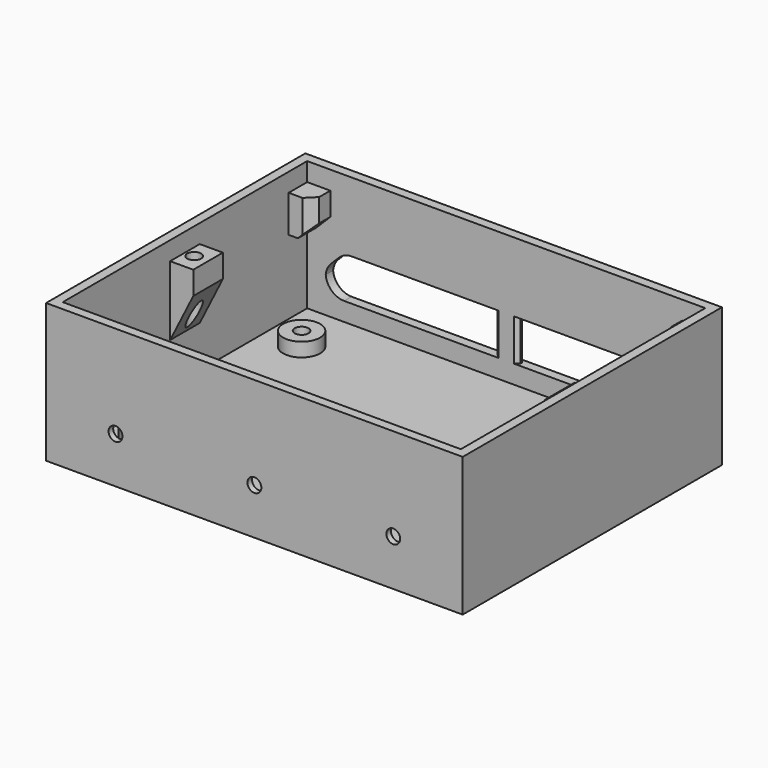
from build123d import *

# Parameters (mm, degrees)
F0_R         = 4
F0_R_2       = 1.5
F1_DEPTH     = 5
F0_W         = 86
F0_H         = 66
F2_DEPTH     = 2
F0_W_2       = 90
F0_H_2       = 70
F3_DEPTH     = 30
F4_R         = 1.5
F5_DEPTH     = 2
F6_R         = 3
F6_R_2       = 1.5
F7_DEPTH     = 0.75
F9_W         = 5
F9_H         = 5
F10_DEPTH    = 8
F11_C1_SIZE  = 3
F11_C2_SIZE  = 3
F11_C3_SIZE  = 3
F11_C4_SIZE  = 3
F12_SIZE     = 2
F13_W        = 78
F13_H        = 9
F14_DEPTH    = 2
F15_SIZE     = 4
F16_T1_DEPTH = 2
F17_W        = 5
F17_H        = 2
F18_DEPTH    = 9
F19_SIZE     = 0.8
F9_H_2       = 8
F9_R         = 1.5
F20_DEPTH    = 15
F21_T4_DEPTH = 59.7965774757
F21_T9_DEPTH = 59.7965774757


# Not quite as in the source:
# - a fillet or chamfer that OpenCascade refuses, or shapes differently, is made with other operations: its cross-section is extruded or revolved along the edge and cut away or added
# - two fillets or chamfers of one size are made in one step


with BuildPart() as f1:
    # F0 (on Top) → F1 (new body)
    with BuildSketch(Plane.XY):
        with Locations((-35, 21.5)):
            Circle(F0_R)
        with Locations((-35, 21.5)):
            Circle(F0_R_2, mode=Mode.SUBTRACT)
    extrude(amount=F1_DEPTH)



with BuildPart() as f1b:
    # F0 (on Top) → F1, piece 2 (new body)
    with BuildSketch(Plane.XY):
        with Locations((35, 21.5)):
            Circle(F0_R)
        with Locations((35, 21.5)):
            Circle(F0_R_2, mode=Mode.SUBTRACT)
    extrude(amount=F1_DEPTH)


with BuildPart() as f1c:
    # F0 (on Top) → F1, piece 3 (new body)
    with BuildSketch(Plane.XY):
        with Locations((35, -21.5)):
            Circle(F0_R)
        with Locations((35, -21.5)):
            Circle(F0_R_2, mode=Mode.SUBTRACT)
    extrude(amount=F1_DEPTH)


with BuildPart() as f1d:
    # F0 (on Top) → F1, piece 4 (new body)
    with BuildSketch(Plane.XY):
        with Locations((-35, -21.5)):
            Circle(F0_R)
        with Locations((-35, -21.5)):
            Circle(F0_R_2, mode=Mode.SUBTRACT)
    extrude(amount=F1_DEPTH)


with BuildPart() as f1_1:
    add(f1.part)

    add(f1b.part)  # F2 merges F1b

    add(f1c.part)  # F2 merges F1c

    add(f1d.part)  # F2 merges F1d
    # F0 (on Top) → F2 (join)
    with BuildSketch(Plane.XY):
        Rectangle(F0_W, F0_H)
        with Locations((-35, -21.5)):
            Circle(F0_R, mode=Mode.SUBTRACT)
        with Locations((35, -21.5)):
            Circle(F0_R, mode=Mode.SUBTRACT)
        with Locations((-35, 21.5)):
            Circle(F0_R, mode=Mode.SUBTRACT)
        with Locations((35, 21.5)):
            Circle(F0_R, mode=Mode.SUBTRACT)
        with Locations((-35, 21.5)):
            Circle(F0_R)
        with Locations((-35, 21.5)):
            Circle(F0_R_2, mode=Mode.SUBTRACT)
        with Locations((35, 21.5)):
            Circle(F0_R_2)
        with Locations((35, -21.5)):
            Circle(F0_R_2)
        with Locations((-35, -21.5)):
            Circle(F0_R_2)
        with Locations((-35, 21.5)):
            Circle(F0_R_2)
    extrude(amount=F2_DEPTH)

    # F0 (on Top) → F3 (join)
    with BuildSketch(Plane.XY):
        Rectangle(F0_W_2, F0_H_2)
        Rectangle(F0_W, F0_H, mode=Mode.SUBTRACT)
    extrude(amount=F3_DEPTH)

    # F4 (on face) → F5 (cut, through all)
    with BuildSketch(Plane.XZ.offset(35)):
        with Locations((-30, 10)):
            Circle(F4_R)
        with Locations((0, 10)):
            Circle(F4_R)
        with Locations((30, 10)):
            Circle(F4_R)
    extrude(amount=-F5_DEPTH, mode=Mode.SUBTRACT)

    # F6 (on face) → F7 (cut)
    with BuildSketch(Plane(origin=(0, -33, 0), x_dir=(-1, 0, 0), z_dir=(0, 1, 0))):
        with Locations((-30, 10)):
            Circle(F6_R)
        with Locations((-30, 10)):
            Circle(F6_R_2, mode=Mode.SUBTRACT)
        with Locations((0, 10)):
            Circle(F6_R)
        with Locations((0, 10)):
            Circle(F6_R_2, mode=Mode.SUBTRACT)
        with Locations((30, 10)):
            Circle(F6_R)
        with Locations((30, 10)):
            Circle(F6_R_2, mode=Mode.SUBTRACT)
    extrude(amount=-F7_DEPTH, mode=Mode.SUBTRACT)

    # F9 (on offset) → F10 (join)
    with BuildSketch(Plane.XY.offset(26)):
        with Locations((40.5, -30.5)):
            Rectangle(F9_W, F9_H)
        with Locations((40.5, 30.5)):
            Rectangle(F9_W, F9_H)
        with Locations((-40.5, -30.5)):
            Rectangle(F9_W, F9_H)
        with Locations((-40.5, 30.5)):
            Rectangle(F9_W, F9_H)
    extrude(amount=-F10_DEPTH)

    # F11: chamfer of 3 on 4 edges, made by hand

    # F11_c1
    f11_c1_edges = [f1_1.edges().sort_by_distance(p)[0] for p in [
        (-38, -30.5, 18),
    ]]
    chamfer(f11_c1_edges, length=F11_C1_SIZE)

    # F11_c2
    f11_c2_edges = [f1_1.edges().sort_by_distance(p)[0] for p in [
        (38, -30.5, 18),
    ]]
    chamfer(f11_c2_edges, length=F11_C2_SIZE)

    # F11_c3
    f11_c3_edges = [f1_1.edges().sort_by_distance(p)[0] for p in [
        (-38, 30.5, 18),
    ]]
    chamfer(f11_c3_edges, length=F11_C3_SIZE)

    # F11_c4
    f11_c4_edges = [f1_1.edges().sort_by_distance(p)[0] for p in [
        (38, 30.5, 18),
    ]]
    chamfer(f11_c4_edges, length=F11_C4_SIZE)

    # F12
    f12_edges = [f1_1.edges().sort_by_distance(p)[0] for p in [
        (-38, 28, 23.5),
        (-38, -28, 23.5),
        (38, -28, 23.5),
        (38, 28, 23.5),
    ]]
    chamfer(f12_edges, length=F12_SIZE)

    # F13 (on face) → F14 (cut, through all)
    with BuildSketch(Plane(origin=(0, 35, 0), x_dir=(-1, 0, 0), z_dir=(0, 1, 0))):
        with Locations((0, 10.5)):
            Rectangle(F13_W, F13_H)
    extrude(amount=-F14_DEPTH, mode=Mode.SUBTRACT)

    # F15
    f15_edges = [f1_1.edges().sort_by_distance(p)[0] for p in [
        (-39, 34, 15),
        (39, 34, 15),
    ]]
    chamfer(f15_edges, length=F15_SIZE)

    # F16: fillet of radius 4 on 6 edges, made by hand

    # F16_s2 → F16_t1 (join)
    with BuildSketch(Plane.XZ.offset(-35)):
        with BuildLine():
            ThreePointArc((-39, 10), (-37.8284271247, 7.1715728753), (-35, 6))
            Line((-35, 6), (-39, 6))
            Line((-39, 6), (-39, 10))
        make_face()
        with BuildLine():
            ThreePointArc((39, 10), (37.8284271247, 7.1715728753), (35, 6))
            Line((35, 6), (39, 6))
            Line((39, 6), (39, 10))
        make_face()
        with BuildLine():
            ThreePointArc((-33.3431457505, 15), (-34.87387948, 14.69551813), (-36.1715728753, 13.8284271247))
            Line((-36.1715728753, 13.8284271247), (-35, 15))
            Line((-35, 15), (-33.3431457505, 15))
        make_face()
        with BuildLine():
            ThreePointArc((33.3431457505, 15), (34.87387948, 14.69551813), (36.1715728753, 13.8284271247))
            Line((36.1715728753, 13.8284271247), (35, 15))
            Line((35, 15), (33.3431457505, 15))
        make_face()
        with BuildLine():
            ThreePointArc((-37.8284271247, 12.1715728753), (-38.69551813, 10.87387948), (-39, 9.3431457505))
            Line((-39, 9.3431457505), (-39, 11))
            Line((-39, 11), (-37.8284271247, 12.1715728753))
        make_face()
        with BuildLine():
            ThreePointArc((37.8284271247, 12.1715728753), (38.69551813, 10.87387948), (39, 9.3431457505))
            Line((39, 9.3431457505), (39, 11))
            Line((39, 11), (37.8284271247, 12.1715728753))
        make_face()
    extrude(amount=F16_T1_DEPTH)

    # F17 (on face) → F18 (join, through all)
    with BuildSketch(Plane(origin=(0, 0, 15), x_dir=(1, 0, 0), z_dir=(0, 0, -1))):
        with Locations((0, -34)):
            Rectangle(F17_W, F17_H)
    extrude(amount=F18_DEPTH)

    # F19
    f19_edges = [f1_1.edges().sort_by_distance(p)[0] for p in [
        (2.5, 35, 10.5),
        (-2.5, 35, 10.5),
        (2.5, 33, 10.5),
        (-2.5, 33, 10.5),
    ]]
    chamfer(f19_edges, length=F19_SIZE)

    # F9 (on offset) → F20 (join)
    with BuildSketch(Plane.XY.offset(26)):
        with Locations((-40.5, 0)):
            Rectangle(F9_W, F9_H_2)
        with Locations((-41, 0)):
            Circle(F9_R, mode=Mode.SUBTRACT)
        with Locations((40.5, 0)):
            Rectangle(F9_W, F9_H_2)
        with Locations((41, 0)):
            Circle(F9_R, mode=Mode.SUBTRACT)
    extrude(amount=-F20_DEPTH)

    # F21: chamfer of 5 x 10 on 2 edges, made by hand


with BuildPart() as f21_tool2:
    # F21_s3 → F21_t4 (new body)
    with BuildSketch(Plane.XZ.offset(-29.8982887379)):
        Polygon((38, 21), (43, 11), (38, 11), align=None)
    extrude(amount=F21_T4_DEPTH)

    split(bisect_by=Plane.YZ.offset(43), keep=Keep.BOTTOM)


with BuildPart() as f1_2:
    add(f1_1.part)

    # F21_t1: cut F21_tool2
    add(f21_tool2.part, mode=Mode.SUBTRACT)


with BuildPart() as f21_tool7:
    # F21_s8 → F21_t9 (new body)
    with BuildSketch(Plane.XZ.offset(29.8982887379)):
        Polygon((-38, 21), (-43, 11), (-38, 11), align=None)
    extrude(amount=-F21_T9_DEPTH)

    split(bisect_by=Plane.YZ.offset(-43), keep=Keep.TOP)


with BuildPart() as f1_3:
    add(f1_2.part)

    # F21_t6: cut F21_tool7
    add(f21_tool7.part, mode=Mode.SUBTRACT)


solid = f1_3.part
